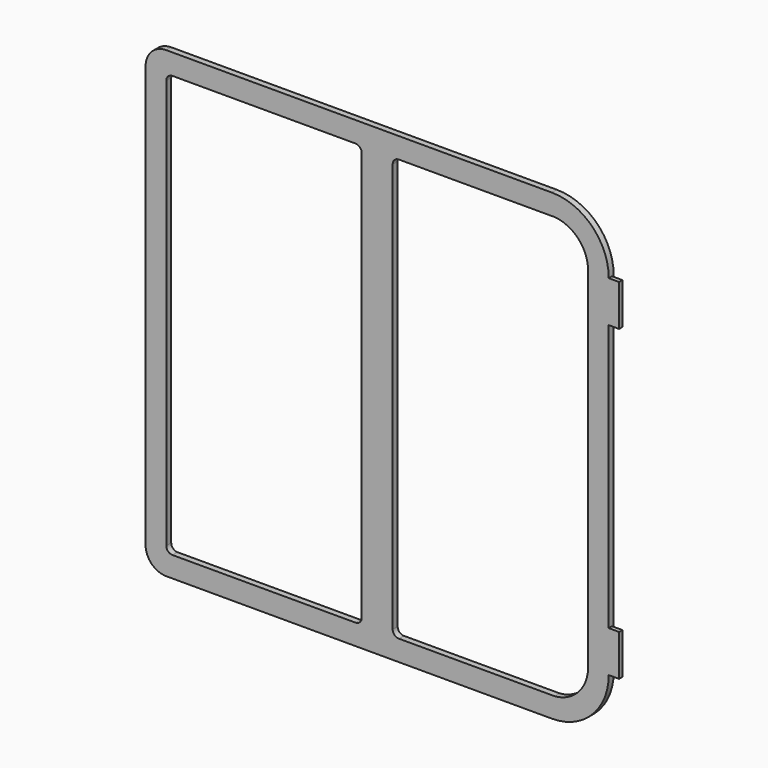
from build123d import *

# Parameters (mm, degrees)
F0_W     = 10
F0_H     = 40
F0_W_2   = 6
F0_W_3   = 14
F0_H_2   = 258
F1_DEPTH = 6
F2_DEPTH = 2


with BuildPart() as f1:
    # F0 (on Front) → F1 (new body)
    with BuildSketch(Plane.XZ):
        with BuildLine():
            Line((185.575712414, 225.5297148285), (-187.424287586, 225.5297148285))
            ThreePointArc((-187.424287586, 225.5297148285), (-201.5664232098, 219.6718504522), (-207.424287586, 205.5297148285))
            Line((-207.424287586, 205.5297148285), (-207.424287586, -202.4702851715))
            ThreePointArc((-207.424287586, -202.4702851715), (-201.5664232098, -216.6124207953), (-187.424287586, -222.4702851715))
            Line((-187.424287586, -222.4702851715), (185.575712414, -222.4702851715))
            ThreePointArc((185.575712414, -222.4702851715), (224.4665853792, -206.3611581368), (240.575712414, -167.4702851715))
            Line((240.575712414, -167.4702851715), (234.575712414, -167.4702851715))
            ThreePointArc((234.575712414, -167.4702851715), (220.2239446921, -202.1185174497), (185.575712414, -216.4702851715))
            Line((185.575712414, -216.4702851715), (-187.424287586, -216.4702851715))
            ThreePointArc((-187.424287586, -216.4702851715), (-197.3237825226, -212.3697801081), (-201.424287586, -202.4702851715))
            Line((-201.424287586, -202.4702851715), (-201.424287586, 205.5297148285))
            ThreePointArc((-201.424287586, 205.5297148285), (-197.3237825226, 215.4292097651), (-187.424287586, 219.5297148285))
            Line((-187.424287586, 219.5297148285), (185.575712414, 219.5297148285))
            ThreePointArc((185.575712414, 219.5297148285), (220.2239446921, 205.1779471066), (234.575712414, 170.5297148285))
            Line((234.575712414, 170.5297148285), (240.575712414, 170.5297148285))
            ThreePointArc((240.575712414, 170.5297148285), (224.4665853792, 209.4205877937), (185.575712414, 225.5297148285))
        make_face()
        with BuildLine():
            Line((220.575712414, 170.5297148285), (234.575712414, 170.5297148285))
            ThreePointArc((234.575712414, 170.5297148285), (220.2239446921, 205.1779471066), (185.575712414, 219.5297148285))
            Line((185.575712414, 219.5297148285), (-187.424287586, 219.5297148285))
            ThreePointArc((-187.424287586, 219.5297148285), (-197.3237825226, 215.4292097651), (-201.424287586, 205.5297148285))
            Line((-201.424287586, 205.5297148285), (-201.424287586, -202.4702851715))
            ThreePointArc((-201.424287586, -202.4702851715), (-197.3237825226, -212.3697801081), (-187.424287586, -216.4702851715))
            Line((-187.424287586, -216.4702851715), (185.575712414, -216.4702851715))
            ThreePointArc((185.575712414, -216.4702851715), (220.2239446921, -202.1185174497), (234.575712414, -167.4702851715))
            Line((234.575712414, -167.4702851715), (220.575712414, -167.4702851715))
            ThreePointArc((220.575712414, -167.4702851715), (211.315135886, -191.295361085), (188.325712414, -202.4702851715))
            Line((188.325712414, -202.4702851715), (37.575712414, -202.4702851715))
            ThreePointArc((37.575712414, -202.4702851715), (33.3330717268, -200.7129258587), (31.575712414, -196.4702851715))
            Line((31.575712414, -196.4702851715), (31.575712414, 199.5297148285))
            ThreePointArc((31.575712414, 199.5297148285), (33.3330717268, 203.7723555156), (37.575712414, 205.5297148285))
            Line((37.575712414, 205.5297148285), (188.325712414, 205.5297148285))
            ThreePointArc((188.325712414, 205.5297148285), (211.315135886, 194.354790742), (220.575712414, 170.5297148285))
        make_face()
        with BuildLine():
            Line((-187.424287586, -196.4702851715), (-187.424287586, 199.5297148285))
            ThreePointArc((-187.424287586, 199.5297148285), (-185.6669282732, 203.7723555156), (-181.424287586, 205.5297148285))
            Line((-181.424287586, 205.5297148285), (-4.424287586, 205.5297148285))
            ThreePointArc((-4.424287586, 205.5297148285), (-0.1816468989, 203.7723555156), (1.575712414, 199.5297148285))
            Line((1.575712414, 199.5297148285), (1.575712414, -196.4702851715))
            ThreePointArc((1.575712414, -196.4702851715), (-0.1816468989, -200.7129258587), (-4.424287586, -202.4702851715))
            Line((-4.424287586, -202.4702851715), (-181.424287586, -202.4702851715))
            ThreePointArc((-181.424287586, -202.4702851715), (-185.6669282732, -200.7129258587), (-187.424287586, -196.4702851715))
        make_face(mode=Mode.SUBTRACT)
        with Locations((245.575712414, 150.5297148285)):
            Rectangle(F0_W, F0_H)
        with Locations((237.575712414, 150.5297148285)):
            Rectangle(F0_W_2, F0_H)
        with Locations((227.575712414, 150.5297148285)):
            Rectangle(F0_W_3, F0_H)
        with Locations((227.575712414, 1.5297148285)):
            Rectangle(F0_W_3, F0_H_2)
        with Locations((237.575712414, 1.5297148285)):
            Rectangle(F0_W_2, F0_H_2)
        with Locations((237.575712414, -147.4702851715)):
            Rectangle(F0_W_2, F0_H)
        with Locations((227.575712414, -147.4702851715)):
            Rectangle(F0_W_3, F0_H)
        with Locations((245.575712414, -147.4702851715)):
            Rectangle(F0_W, F0_H)
    extrude(amount=F1_DEPTH)

    # F0 (on Front) → F2 (cut)
    with BuildSketch(Plane.XZ):
        with Locations((245.575712414, 150.5297148285)):
            Rectangle(F0_W, F0_H)
        with Locations((245.575712414, -147.4702851715)):
            Rectangle(F0_W, F0_H)
    extrude(amount=F2_DEPTH, mode=Mode.SUBTRACT)


solid = f1.part
